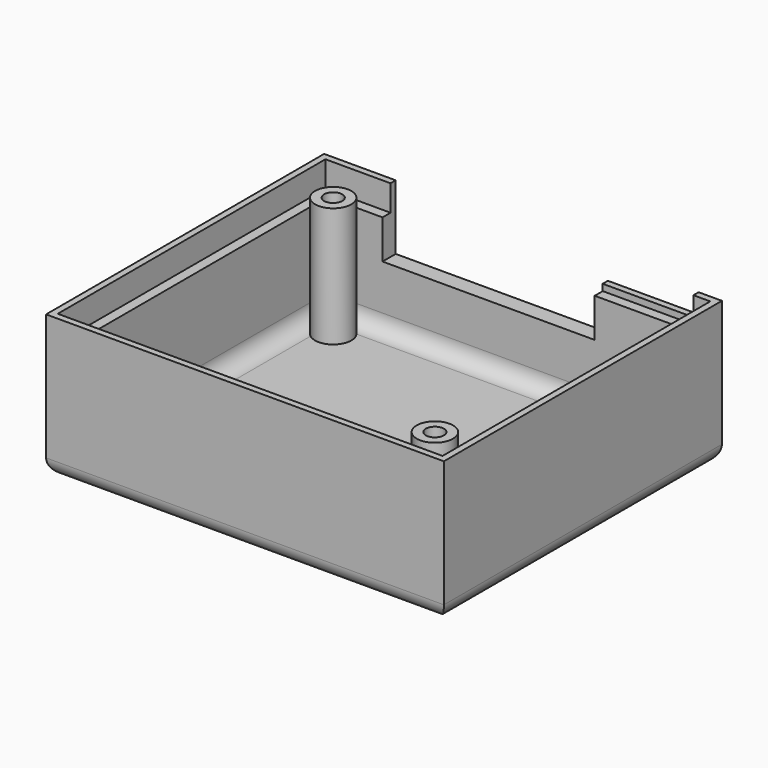
from build123d import *

# Parameters (mm, degrees)
F0_W        = 56.3
F0_H        = 48.55
F0_R        = 2.8
F1_DEPTH    = 2.5
F0_W_2      = 59.4
F0_H_2      = 51.65
F2_DEPTH    = 18
F0_W_3      = 61.4
F0_H_3      = 53.65
F3_DEPTH    = 22
F0_R_2      = 1.4
F4_DEPTH    = 21
F5_DEPTH    = 15
F6_T1_DEPTH = 48.55
F6_T3_DEPTH = 56.3
F6_T5_DEPTH = 73.9
F6_T7_DEPTH = 66.15
F7_W        = 32.75
F7_H        = 1
F7_H_2      = 1.55
F8_DEPTH    = 10
F7_W_2      = 14
F9_DEPTH    = 3


# Not quite as in the source:
# - a fillet or chamfer that OpenCascade refuses, or shapes differently, is made with other operations: its cross-section is extruded or revolved along the edge and cut away or added


with BuildPart() as f1:
    # F0 (on Top) → F1 (new body)
    with BuildSketch(Plane.XY):
        Rectangle(F0_W, F0_H)
        with Locations((23.88, -20.035)):
            Circle(F0_R, mode=Mode.SUBTRACT)
        with Locations((-23.91, 20.085)):
            Circle(F0_R, mode=Mode.SUBTRACT)
    extrude(amount=F1_DEPTH)

    # F0 (on Top) → F2 (join)
    with BuildSketch(Plane.XY):
        Rectangle(F0_W_2, F0_H_2)
        Rectangle(F0_W, F0_H, mode=Mode.SUBTRACT)
    extrude(amount=F2_DEPTH)

    # F0 (on Top) → F3 (join)
    with BuildSketch(Plane.XY):
        Rectangle(F0_W_3, F0_H_3)
        Rectangle(F0_W_2, F0_H_2, mode=Mode.SUBTRACT)
    extrude(amount=F3_DEPTH)

    # F0 (on Top) → F4 (join)
    with BuildSketch(Plane.XY):
        with Locations((-23.91, 20.085)):
            Circle(F0_R)
        with Locations((-23.91, 20.085)):
            Circle(F0_R_2, mode=Mode.SUBTRACT)
        with Locations((23.88, -20.035)):
            Circle(F0_R)
        with Locations((23.88, -20.035)):
            Circle(F0_R_2, mode=Mode.SUBTRACT)
    extrude(amount=F4_DEPTH)

    # F0 (on Top) → F5 (join)
    with BuildSketch(Plane.XY):
        with Locations((23.88, -20.035)):
            Circle(F0_R_2)
        with Locations((-23.91, 20.085)):
            Circle(F0_R_2)
    extrude(amount=F5_DEPTH)

    # F6: fillet of radius 2.5 on 8 edges, made by hand

    # F6_s2 → F6_t1 (join)
    with BuildSketch(Plane.XZ.offset(-24.275)):
        with BuildLine():
            ThreePointArc((28.15, 5), (27.417766953, 3.232233047), (25.65, 2.5))
            Line((25.65, 2.5), (28.15, 2.5))
            Line((28.15, 2.5), (28.15, 5))
        make_face()
        with BuildLine():
            ThreePointArc((-28.15, 5), (-27.417766953, 3.232233047), (-25.65, 2.5))
            Line((-25.65, 2.5), (-28.15, 2.5))
            Line((-28.15, 2.5), (-28.15, 5))
        make_face()
    extrude(amount=F6_T1_DEPTH)

    # F6_s4 → F6_t3 (join)
    with BuildSketch(Plane.YZ.offset(-28.15)):
        with BuildLine():
            ThreePointArc((24.275, 5), (23.542766953, 3.232233047), (21.775, 2.5))
            Line((21.775, 2.5), (24.275, 2.5))
            Line((24.275, 2.5), (24.275, 5))
        make_face()
        with BuildLine():
            ThreePointArc((-24.275, 5), (-23.542766953, 3.232233047), (-21.775, 2.5))
            Line((-21.775, 2.5), (-24.275, 2.5))
            Line((-24.275, 2.5), (-24.275, 5))
        make_face()
    extrude(amount=F6_T3_DEPTH)

    # F6_s6 → F6_t5 (cut)
    with BuildSketch(Plane.YZ.offset(-36.95)):
        with BuildLine():
            ThreePointArc((-24.325, 0), (-26.092766953, 0.732233047), (-26.825, 2.5))
            Line((-26.825, 2.5), (-26.825, 0))
            Line((-26.825, 0), (-24.325, 0))
        make_face()
        with BuildLine():
            ThreePointArc((24.325, 0), (26.092766953, 0.732233047), (26.825, 2.5))
            Line((26.825, 2.5), (26.825, 0))
            Line((26.825, 0), (24.325, 0))
        make_face()
    extrude(amount=F6_T5_DEPTH, mode=Mode.SUBTRACT)

    # F6_s8 → F6_t7 (cut)
    with BuildSketch(Plane.XZ.offset(-33.075)):
        with BuildLine():
            ThreePointArc((28.2, 0), (29.967766953, 0.732233047), (30.7, 2.5))
            Line((30.7, 2.5), (30.7, 0))
            Line((30.7, 0), (28.2, 0))
        make_face()
        with BuildLine():
            ThreePointArc((-28.2, 0), (-29.967766953, 0.732233047), (-30.7, 2.5))
            Line((-30.7, 2.5), (-30.7, 0))
            Line((-30.7, 0), (-28.2, 0))
        make_face()
    extrude(amount=F6_T7_DEPTH, mode=Mode.SUBTRACT)

    # F7 (on face) → F8 (cut)
    with BuildSketch(Plane.XY.offset(22)):
        with Locations((-3.275, 26.325)):
            Rectangle(F7_W, F7_H)
        with Locations((-3.275, 25.05)):
            Rectangle(F7_W, F7_H_2)
    extrude(amount=-F8_DEPTH, mode=Mode.SUBTRACT)

    # F7 (on face) → F9 (cut)
    with BuildSketch(Plane.XY.offset(22)):
        with Locations((20.1, 26.325)):
            Rectangle(F7_W_2, F7_H)
        with Locations((20.1, 25.05)):
            Rectangle(F7_W_2, F7_H_2)
    extrude(amount=-F9_DEPTH, mode=Mode.SUBTRACT)


solid = f1.part
